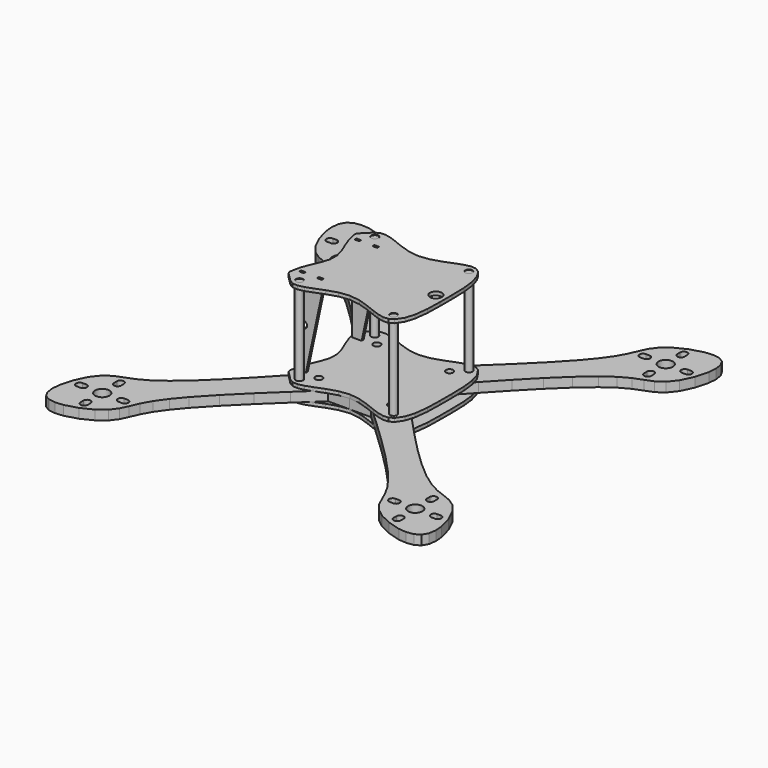
from build123d import *

# Parameters (mm, degrees)
F0_R      = 1.5
F0_R_2    = 3
F1_DEPTH  = 4
F3_DEPTH  = 4
F9_R      = 1.5
F10_DEPTH = 1.5
F12_R     = 1.5
F12_W     = 2
F12_H     = 1
F13_DEPTH = 1.5
F15_R     = 1.5
F15_W     = 2
F15_H     = 1
F15_R_2   = 2.5
F16_DEPTH = 1.5
F18_R     = 1.5
F19_DEPTH = 1
F21_DEPTH = 1
F23_R     = 1.5106239122
F24_DEPTH = 41.8
F23_R_2   = 1.5194161775
F23_R_3   = 1.519414421
F23_R_4   = 1.4934796866


# Not quite as in the source:
# - ends of sketch curves that miss each other by under 0.0002 mm in the source are joined


with BuildPart() as f1:
    # F0 (on Top) → F1 (new body)
    with BuildSketch(Plane.XY):
        Polygon((14.588631, -22.89682), (22.280861, -31.264773), (22.280861, -40.264773), (40.280861, -40.264773), (40.280861, -22.264773), (31.280861, -22.264773), (22.197863, -13.784713), (13.473396, -5.476525), (5.46599, 2.48792), (-1.465825, 9.93675), (-5.626846, 14.932085), (-8.891406, 19.497675), (-11.146676, 23.572215), (-12.706403, 27.176122), (-14.241022, 30.398156), (-16.431942, 33.329176), (-19.919393, 36.045885), (-24.80687, 38.450624), (-30.130665, 39.971349), (-33.488305, 40.264773), (-36.388928, 39.821389), (-38.572162, 38.503632), (-39.84702, 36.246807), (-40.280861, 33.257523), (-40.001152, 29.805519), (-38.522527, 24.349964), (-36.155436, 19.370567), (-33.323541, 15.755781), (-30.226835, 13.645808), (-26.791513, 12.264865), (-22.927057, 10.781282), (-18.549265, 8.401879), (-13.663209, 4.878131), (-7.22952, -0.641392), (-0.292414, -7.300286), (7.022254, -14.81371), align=None)
        with Locations((25.030861, -25.014773)):
            Circle(F0_R, mode=Mode.SUBTRACT)
        with Locations((20.513094, -20.497006)):
            Circle(F0_R, mode=Mode.SUBTRACT)
        with BuildLine():
            ThreePointArc((-26.922394, 17.438495), (-25.422394, 18.938495), (-23.922394, 17.438495))
            Line((-23.922394, 17.438495), (-23.922394, 15.938495))
            ThreePointArc((-23.922394, 15.938495), (-25.422394, 14.438495), (-26.922394, 15.938495))
            Line((-26.922394, 15.938495), (-26.922394, 17.438495))
        make_face(mode=Mode.SUBTRACT)
        with BuildLine():
            ThreePointArc((-34.922394, 23.938495), (-36.422394, 25.438495), (-34.922394, 26.938495))
            Line((-34.922394, 26.938495), (-33.422394, 26.938495))
            ThreePointArc((-33.422394, 26.938495), (-31.922394, 25.438495), (-33.422394, 23.938495))
            Line((-33.422394, 23.938495), (-34.922394, 23.938495))
        make_face(mode=Mode.SUBTRACT)
        with Locations((-25.427944, 25.444032)):
            Circle(F0_R_2, mode=Mode.SUBTRACT)
        with BuildLine():
            ThreePointArc((-23.922394, 33.438495), (-25.422394, 31.938495), (-26.922394, 33.438495))
            Line((-26.922394, 33.438495), (-26.922394, 34.938495))
            ThreePointArc((-26.922394, 34.938495), (-25.422394, 36.438495), (-23.922394, 34.938495))
            Line((-23.922394, 34.938495), (-23.922394, 33.438495))
        make_face(mode=Mode.SUBTRACT)
        with BuildLine():
            ThreePointArc((-15.922394, 26.938495), (-14.422394, 25.438495), (-15.922394, 23.938495))
            Line((-15.922394, 23.938495), (-17.422394, 23.938495))
            ThreePointArc((-17.422394, 23.938495), (-18.922394, 25.438495), (-17.422394, 26.938495))
            Line((-17.422394, 26.938495), (-15.922394, 26.938495))
        make_face(mode=Mode.SUBTRACT)
    extrude(amount=F1_DEPTH)


with BuildPart() as f1_1:
    # F2: moved
    add(f1.part.moved(Location((-40.3, 40.3, 0))))


with BuildPart() as f3:
    # F0 (on Top) → F3 (new body)
    with BuildSketch(Plane.XY):
        Polygon((14.588631, -22.89682), (22.280861, -31.264773), (22.280861, -40.264773), (40.280861, -40.264773), (40.280861, -22.264773), (31.280861, -22.264773), (22.197863, -13.784713), (13.473396, -5.476525), (5.46599, 2.48792), (-1.465825, 9.93675), (-5.626846, 14.932085), (-8.891406, 19.497675), (-11.146676, 23.572215), (-12.706403, 27.176122), (-14.241022, 30.398156), (-16.431942, 33.329176), (-19.919393, 36.045885), (-24.80687, 38.450624), (-30.130665, 39.971349), (-33.488305, 40.264773), (-36.388928, 39.821389), (-38.572162, 38.503632), (-39.84702, 36.246807), (-40.280861, 33.257523), (-40.001152, 29.805519), (-38.522527, 24.349964), (-36.155436, 19.370567), (-33.323541, 15.755781), (-30.226835, 13.645808), (-26.791513, 12.264865), (-22.927057, 10.781282), (-18.549265, 8.401879), (-13.663209, 4.878131), (-7.22952, -0.641392), (-0.292414, -7.300286), (7.022254, -14.81371), align=None)
        with Locations((25.030861, -25.014773)):
            Circle(F0_R, mode=Mode.SUBTRACT)
        with Locations((20.513094, -20.497006)):
            Circle(F0_R, mode=Mode.SUBTRACT)
        with BuildLine():
            ThreePointArc((-26.922394, 17.438495), (-25.422394, 18.938495), (-23.922394, 17.438495))
            Line((-23.922394, 17.438495), (-23.922394, 15.938495))
            ThreePointArc((-23.922394, 15.938495), (-25.422394, 14.438495), (-26.922394, 15.938495))
            Line((-26.922394, 15.938495), (-26.922394, 17.438495))
        make_face(mode=Mode.SUBTRACT)
        with BuildLine():
            ThreePointArc((-34.922394, 23.938495), (-36.422394, 25.438495), (-34.922394, 26.938495))
            Line((-34.922394, 26.938495), (-33.422394, 26.938495))
            ThreePointArc((-33.422394, 26.938495), (-31.922394, 25.438495), (-33.422394, 23.938495))
            Line((-33.422394, 23.938495), (-34.922394, 23.938495))
        make_face(mode=Mode.SUBTRACT)
        with Locations((-25.427944, 25.444032)):
            Circle(F0_R_2, mode=Mode.SUBTRACT)
        with BuildLine():
            ThreePointArc((-23.922394, 33.438495), (-25.422394, 31.938495), (-26.922394, 33.438495))
            Line((-26.922394, 33.438495), (-26.922394, 34.938495))
            ThreePointArc((-26.922394, 34.938495), (-25.422394, 36.438495), (-23.922394, 34.938495))
            Line((-23.922394, 34.938495), (-23.922394, 33.438495))
        make_face(mode=Mode.SUBTRACT)
        with BuildLine():
            ThreePointArc((-15.922394, 26.938495), (-14.422394, 25.438495), (-15.922394, 23.938495))
            Line((-15.922394, 23.938495), (-17.422394, 23.938495))
            ThreePointArc((-17.422394, 23.938495), (-18.922394, 25.438495), (-17.422394, 26.938495))
            Line((-17.422394, 26.938495), (-15.922394, 26.938495))
        make_face(mode=Mode.SUBTRACT)
    extrude(amount=F3_DEPTH)


with BuildPart() as f4_1:
    # F4: instance of F3
    add(f3.part.mirror(Plane.XZ))


with BuildPart() as f4_1_1:
    # F5: moved
    add(f4_1.part.moved(Location((-40.3, -40.3, 0))))


with BuildPart() as f7_1:
    # F7: instance of F1
    add(f1_1.part.mirror(Plane.YZ))


with BuildPart() as f8_1:
    # F8: instance of F7_1
    add(f7_1.part.mirror(Plane.XZ))


with BuildPart() as f10:
    # F9 (on Top) → F10 (new body)
    with BuildSketch(Plane.XY):
        with BuildLine():
            Line((-25.3842725429, -18.2968425442), (-21.776806, -21.90469))
            ThreePointArc((-21.776806, -21.90469), (-21.7695847524, -21.9118754367), (-21.7623269391, -21.9190239378))
            Line((-21.7623269391, -21.9190239378), (-20.001088, -22.921175))
            Line((-20.001088, -22.921175), (-17.861866, -23.035324))
            Line((-17.861866, -23.035324), (-15.372177, -22.484303))
            Line((-15.372177, -22.484303), (-12.607263, -21.500754))
            Line((-12.607263, -21.500754), (-8.588488, -19.927774))
            Line((-8.588488, -19.927774), (-4.3106, -18.572828))
            Line((-4.3106, -18.572828), (0.094871, -17.999903))
            Line((0.094871, -17.999903), (4.497054, -18.584621))
            Line((4.497054, -18.584621), (8.767715, -19.949316))
            Line((8.767715, -19.949316), (12.779279, -21.528046))
            Line((12.779279, -21.528046), (15.541174, -22.512101))
            Line((15.541174, -22.512101), (18.031746, -23.059449))
            Line((18.031746, -23.059449), (20.197174, -22.931331))
            Line((20.197174, -22.931331), (21.983635, -21.88899))
            Line((21.983635, -21.88899), (23.940328, -18.98249))
            Line((23.940328, -18.98249), (25.122837, -15.218566))
            Line((25.122837, -15.218566), (25.815172, -9.515305))
            Line((25.815172, -9.515305), (25.969817, -3.186776))
            Line((25.969817, -3.186776), (25.969969, 3.339753))
            Line((25.969969, 3.339753), (25.807978, 9.644786))
            Line((25.807978, 9.644786), (25.256208, 14.514056))
            Line((25.256208, 14.514056), (24.06386, 18.675831))
            Line((24.06386, 18.675831), (21.985337, 21.878655))
            ThreePointArc((21.985337, 21.878655), (21.9798580505, 21.8841874891), (21.9743579768, 21.8896989767))
            Line((21.9743579768, 21.8896989767), (20.209215, 22.909511))
            Line((20.209215, 22.909511), (18.056913, 23.026143))
            Line((18.056913, 23.026143), (15.568049, 22.474392))
            Line((15.568049, 22.474392), (12.802409, 21.490951))
            Line((12.802409, 21.490951), (8.781129, 19.919049))
            Line((8.781129, 19.919049), (4.50007, 18.565781))
            Line((4.50007, 18.565781), (0.091958, 17.994625))
            Line((0.091958, 17.994625), (-4.31142, 18.580902))
            Line((-4.31142, 18.580902), (-8.582017, 19.946966))
            Line((-8.582017, 19.946966), (-12.592724, 21.526836))
            Line((-12.592724, 21.526836), (-15.353738, 22.511578))
            Line((-15.353738, 22.511578), (-17.843441, 23.059449))
            Line((-17.843441, 23.059449), (-19.987611, 22.937283))
            Line((-19.987611, 22.937283), (-21.761576, 21.921992))
            ThreePointArc((-21.761576, 21.921992), (-21.7690321095, 21.9146523137), (-21.7764495624, 21.9072735624))
            Line((-21.7764495624, 21.9072735624), (-25.300048, 18.383676))
            ThreePointArc((-25.300048, 18.383676), (-25.7704478547, 17.6389622754), (-25.8752922762, 16.7643869715))
            Line((-25.8752922762, 16.7643869715), (-24.974945, 12.734506))
            Line((-24.974945, 12.734506), (-23.49499, 8.878377))
            Line((-23.49499, 8.878377), (-21.991471, 5.171737))
            Line((-21.991471, 5.171737), (-21.020436, 1.590323))
            Line((-21.020436, 1.590323), (-21.107345, -1.893192))
            Line((-21.107345, -1.893192), (-22.181047, -5.300749))
            Line((-22.181047, -5.300749), (-23.708361, -8.823601))
            Line((-23.708361, -8.823601), (-25.149676, -12.591593))
            Line((-25.149676, -12.591593), (-25.965377, -16.734569))
            Line((-25.965377, -16.734569), (-25.968026, -16.794603))
            ThreePointArc((-25.968026, -16.794603), (-25.8343859413, -17.606587539), (-25.3851102659, -18.2960292498))
            Line((-25.3851102659, -18.2960292498), (-25.3842725429, -18.2968425442))
        make_face()
        with Locations((-19.630301, -19.80957)):
            Circle(F9_R, mode=Mode.SUBTRACT)
        with Locations((-15.155452, -15.249903)):
            Circle(F9_R, mode=Mode.SUBTRACT)
        with Locations((19.862315, -19.76767)):
            Circle(F9_R, mode=Mode.SUBTRACT)
        with Locations((15.344548, -15.249903)):
            Circle(F9_R, mode=Mode.SUBTRACT)
        with Locations((-15.155452, 15.250097)):
            Circle(F9_R, mode=Mode.SUBTRACT)
        with Locations((-19.673219, 19.767864)):
            Circle(F9_R, mode=Mode.SUBTRACT)
        with Locations((15.344548, 15.250097)):
            Circle(F9_R, mode=Mode.SUBTRACT)
        with Locations((19.862315, 19.767864)):
            Circle(F9_R, mode=Mode.SUBTRACT)
    extrude(amount=F10_DEPTH)


with BuildPart() as f10_1:
    # F11: moved
    add(f10.part.moved(Location((0, 0, -1.5))))


with BuildPart() as f13:
    # F12 (on Top) → F13 (new body)
    with BuildSketch(Plane.XY):
        with BuildLine():
            Line((-25.3842725429, -18.2968425442), (-21.776806, -21.90469))
            ThreePointArc((-21.776806, -21.90469), (-21.7695847524, -21.9118754367), (-21.7623269391, -21.9190239378))
            Line((-21.7623269391, -21.9190239378), (-20.001088, -22.921175))
            Line((-20.001088, -22.921175), (-17.861866, -23.035324))
            Line((-17.861866, -23.035324), (-15.372177, -22.484303))
            Line((-15.372177, -22.484303), (-12.607263, -21.500754))
            Line((-12.607263, -21.500754), (-8.588488, -19.927774))
            Line((-8.588488, -19.927774), (-4.3106, -18.572828))
            Line((-4.3106, -18.572828), (0.094871, -17.999903))
            Line((0.094871, -17.999903), (4.497054, -18.584621))
            Line((4.497054, -18.584621), (8.767715, -19.949316))
            Line((8.767715, -19.949316), (12.779279, -21.528046))
            Line((12.779279, -21.528046), (15.541174, -22.512101))
            Line((15.541174, -22.512101), (18.031746, -23.059449))
            Line((18.031746, -23.059449), (20.197174, -22.931331))
            Line((20.197174, -22.931331), (21.983635, -21.88899))
            Line((21.983635, -21.88899), (23.940328, -18.98249))
            Line((23.940328, -18.98249), (25.122837, -15.218566))
            Line((25.122837, -15.218566), (25.815172, -9.515305))
            Line((25.815172, -9.515305), (25.969817, -3.186776))
            Line((25.969817, -3.186776), (25.969969, 3.339753))
            Line((25.969969, 3.339753), (25.807978, 9.644786))
            Line((25.807978, 9.644786), (25.256208, 14.514056))
            Line((25.256208, 14.514056), (24.06386, 18.675831))
            Line((24.06386, 18.675831), (21.985337, 21.878655))
            ThreePointArc((21.985337, 21.878655), (21.9798580505, 21.8841874891), (21.9743579768, 21.8896989767))
            Line((21.9743579768, 21.8896989767), (20.209215, 22.909511))
            Line((20.209215, 22.909511), (18.056913, 23.026143))
            Line((18.056913, 23.026143), (15.568049, 22.474392))
            Line((15.568049, 22.474392), (12.802409, 21.490951))
            Line((12.802409, 21.490951), (8.781129, 19.919049))
            Line((8.781129, 19.919049), (4.50007, 18.565781))
            Line((4.50007, 18.565781), (0.091958, 17.994625))
            Line((0.091958, 17.994625), (-4.31142, 18.580902))
            Line((-4.31142, 18.580902), (-8.582017, 19.946966))
            Line((-8.582017, 19.946966), (-12.592724, 21.526836))
            Line((-12.592724, 21.526836), (-15.353738, 22.511578))
            Line((-15.353738, 22.511578), (-17.843441, 23.059449))
            Line((-17.843441, 23.059449), (-19.987611, 22.937283))
            Line((-19.987611, 22.937283), (-21.761576, 21.921992))
            ThreePointArc((-21.761576, 21.921992), (-21.7690321095, 21.9146523137), (-21.7764495624, 21.9072735624))
            Line((-21.7764495624, 21.9072735624), (-25.300048, 18.383676))
            ThreePointArc((-25.300048, 18.383676), (-25.7704478547, 17.6389622754), (-25.8752922762, 16.7643869715))
            Line((-25.8752922762, 16.7643869715), (-24.974945, 12.734506))
            Line((-24.974945, 12.734506), (-23.49499, 8.878377))
            Line((-23.49499, 8.878377), (-21.991471, 5.171737))
            Line((-21.991471, 5.171737), (-21.020436, 1.590323))
            Line((-21.020436, 1.590323), (-21.107345, -1.893192))
            Line((-21.107345, -1.893192), (-22.181047, -5.300749))
            Line((-22.181047, -5.300749), (-23.708361, -8.823601))
            Line((-23.708361, -8.823601), (-25.149676, -12.591593))
            Line((-25.149676, -12.591593), (-25.965377, -16.734569))
            Line((-25.965377, -16.734569), (-25.968026, -16.794603))
            ThreePointArc((-25.968026, -16.794603), (-25.8343859413, -17.606587539), (-25.3851102659, -18.2960292498))
            Line((-25.3851102659, -18.2960292498), (-25.3842725429, -18.2968425442))
        make_face()
        with Locations((-19.630301, -19.80957)):
            Circle(F12_R, mode=Mode.SUBTRACT)
        with Locations((-22.655452, -14.499902)):
            Rectangle(F12_W, F12_H, mode=Mode.SUBTRACT)
        with Locations((-15.155452, -15.249903)):
            Circle(F12_R, mode=Mode.SUBTRACT)
        with Locations((19.862315, -19.76767)):
            Circle(F12_R, mode=Mode.SUBTRACT)
        with Locations((15.344548, -15.249903)):
            Circle(F12_R, mode=Mode.SUBTRACT)
        with Locations((-22.655452, 14.600097)):
            Rectangle(F12_W, F12_H, mode=Mode.SUBTRACT)
        with Locations((-15.155452, 15.250097)):
            Circle(F12_R, mode=Mode.SUBTRACT)
        with Locations((-19.673219, 19.767864)):
            Circle(F12_R, mode=Mode.SUBTRACT)
        with Locations((15.344548, 15.250097)):
            Circle(F12_R, mode=Mode.SUBTRACT)
        with Locations((19.862315, 19.767864)):
            Circle(F12_R, mode=Mode.SUBTRACT)
    extrude(amount=F13_DEPTH)


with BuildPart() as f13_1:
    # F14: moved
    add(f13.part.moved(Location((0, 0, 4))))


with BuildPart() as f16:
    # F15 (on Top) → F16 (new body)
    with BuildSketch(Plane.XY):
        with BuildLine():
            Line((-25.3842725429, -18.2968425442), (-21.776806, -21.90469))
            ThreePointArc((-21.776806, -21.90469), (-21.7695847524, -21.9118754367), (-21.7623269391, -21.9190239378))
            Line((-21.7623269391, -21.9190239378), (-20.001088, -22.921175))
            Line((-20.001088, -22.921175), (-17.861866, -23.035324))
            Line((-17.861866, -23.035324), (-15.372177, -22.484303))
            Line((-15.372177, -22.484303), (-12.607263, -21.500754))
            Line((-12.607263, -21.500754), (-8.588488, -19.927774))
            Line((-8.588488, -19.927774), (-4.3106, -18.572828))
            Line((-4.3106, -18.572828), (0.094871, -17.999903))
            Line((0.094871, -17.999903), (4.497054, -18.584621))
            Line((4.497054, -18.584621), (8.767715, -19.949316))
            Line((8.767715, -19.949316), (12.779279, -21.528046))
            Line((12.779279, -21.528046), (15.541174, -22.512101))
            Line((15.541174, -22.512101), (18.031746, -23.059449))
            Line((18.031746, -23.059449), (20.197174, -22.931331))
            Line((20.197174, -22.931331), (21.983635, -21.88899))
            Line((21.983635, -21.88899), (23.940328, -18.98249))
            Line((23.940328, -18.98249), (25.122837, -15.218566))
            Line((25.122837, -15.218566), (25.815172, -9.515305))
            Line((25.815172, -9.515305), (25.969817, -3.186776))
            Line((25.969817, -3.186776), (25.969969, 3.339753))
            Line((25.969969, 3.339753), (25.807978, 9.644786))
            Line((25.807978, 9.644786), (25.256208, 14.514056))
            Line((25.256208, 14.514056), (24.06386, 18.675831))
            Line((24.06386, 18.675831), (22.2375132143, 21.6685608029))
            Line((22.2375132143, 21.6685608029), (20.209215, 22.909511))
            Line((20.209215, 22.909511), (18.056913, 23.026143))
            Line((18.056913, 23.026143), (15.568049, 22.474392))
            Line((15.568049, 22.474392), (12.802409, 21.490951))
            Line((12.802409, 21.490951), (8.781129, 19.919049))
            Line((8.781129, 19.919049), (4.50007, 18.565781))
            Line((4.50007, 18.565781), (0.091958, 17.994625))
            Line((0.091958, 17.994625), (-4.31142, 18.580902))
            Line((-4.31142, 18.580902), (-8.582017, 19.946966))
            Line((-8.582017, 19.946966), (-12.592724, 21.526836))
            Line((-12.592724, 21.526836), (-15.353738, 22.511578))
            Line((-15.353738, 22.511578), (-17.843441, 23.059449))
            Line((-17.843441, 23.059449), (-19.987611, 22.937283))
            Line((-19.987611, 22.937283), (-21.761576, 21.921992))
            ThreePointArc((-21.761576, 21.921992), (-21.7690321095, 21.9146523137), (-21.7764495624, 21.9072735624))
            Line((-21.7764495624, 21.9072735624), (-25.300048, 18.383676))
            ThreePointArc((-25.300048, 18.383676), (-25.7704478547, 17.6389622754), (-25.8752922762, 16.7643869715))
            Line((-25.8752922762, 16.7643869715), (-24.974945, 12.734506))
            Line((-24.974945, 12.734506), (-23.49499, 8.878377))
            Line((-23.49499, 8.878377), (-21.991471, 5.171737))
            Line((-21.991471, 5.171737), (-21.020436, 1.590323))
            Line((-21.020436, 1.590323), (-21.107345, -1.893192))
            Line((-21.107345, -1.893192), (-22.181047, -5.300749))
            Line((-22.181047, -5.300749), (-23.708361, -8.823601))
            Line((-23.708361, -8.823601), (-25.149676, -12.591593))
            Line((-25.149676, -12.591593), (-25.965377, -16.734569))
            Line((-25.965377, -16.734569), (-25.968026, -16.794603))
            ThreePointArc((-25.968026, -16.794603), (-25.8343859413, -17.606587539), (-25.3851102659, -18.2960292498))
            Line((-25.3851102659, -18.2960292498), (-25.3842725429, -18.2968425442))
        make_face()
        with Locations((-19.630301, -19.80957)):
            Circle(F15_R, mode=Mode.SUBTRACT)
        with Locations((-22.655452, -14.499902)):
            Rectangle(F15_W, F15_H, mode=Mode.SUBTRACT)
        with Locations((-15.155479, -14.499902)):
            Rectangle(F15_W, F15_H, mode=Mode.SUBTRACT)
        with Locations((19.862315, -19.76767)):
            Circle(F15_R, mode=Mode.SUBTRACT)
        with Locations((-22.655452, 14.600097)):
            Rectangle(F15_W, F15_H, mode=Mode.SUBTRACT)
        with Locations((-15.155479, 14.600097)):
            Rectangle(F15_W, F15_H, mode=Mode.SUBTRACT)
        with Locations((-19.673219, 19.767864)):
            Circle(F15_R, mode=Mode.SUBTRACT)
        with Locations((21.776255, 9.7e-05)):
            Circle(F15_R_2, mode=Mode.SUBTRACT)
        with Locations((19.862315, 19.767864)):
            Circle(F15_R, mode=Mode.SUBTRACT)
    extrude(amount=F16_DEPTH)


with BuildPart() as f16_1:
    # F17: moved
    add(f16.part.moved(Location((0, 0, 40.5))))


with BuildPart() as f19:
    # F18 (on Front) → F19 (new body)
    with BuildSketch(Plane.XZ):
        Polygon((-4.75, 17.5), (-5.75, 17.5), (-5.75, -17.5), (-4.75, -17.5), (-4.75, -18.5), (-2.75, -18.5), (-2.75, -17.5), (-1.75, -17.5), (5.75, 17.5), (4.75, 17.5), (4.75, 18.5), (2.75, 18.5), (2.75, 17.5), (-2.75, 17.5), (-2.75, 18.5), (-4.75, 18.5), align=None)
        with Locations((-2.75, 0)):
            Circle(F18_R, mode=Mode.SUBTRACT)
    extrude(amount=F19_DEPTH)


with BuildPart() as f19_1:
    # F20: moved
    add(f19.part.moved(Location((-19.03, -14.04, 23.01))))


with BuildPart() as f21:
    # F18 (on Front) → F21 (new body)
    with BuildSketch(Plane.XZ):
        Polygon((-4.75, 17.5), (-5.75, 17.5), (-5.75, -17.5), (-4.75, -17.5), (-4.75, -18.5), (-2.75, -18.5), (-2.75, -17.5), (-1.75, -17.5), (5.75, 17.5), (4.75, 17.5), (4.75, 18.5), (2.75, 18.5), (2.75, 17.5), (-2.75, 17.5), (-2.75, 18.5), (-4.75, 18.5), align=None)
        with Locations((-2.75, 0)):
            Circle(F18_R, mode=Mode.SUBTRACT)
    extrude(amount=F21_DEPTH)


with BuildPart() as f21_1:
    # F22: moved
    add(f21.part.moved(Location((-18.9, 15.1, 23.03))))


with BuildPart() as f24:
    # F23 (on Top) → F24 (new body)
    with BuildSketch(Plane.XY):
        with Locations((-19.7049248964, -19.8188405484)):
            Circle(F23_R)
    extrude(amount=F24_DEPTH)


with BuildPart() as f24b:
    # F23 (on Top) → F24, piece 2 (new body)
    with BuildSketch(Plane.XY):
        with Locations((19.7811666876, -19.7767019272)):
            Circle(F23_R_2)
    extrude(amount=F24_DEPTH)


with BuildPart() as f24c:
    # F23 (on Top) → F24, piece 3 (new body)
    with BuildSketch(Plane.XY):
        with Locations((19.8654476553, 19.7515301406)):
            Circle(F23_R_3)
    extrude(amount=F24_DEPTH)


with BuildPart() as f24d:
    # F23 (on Top) → F24, piece 4 (new body)
    with BuildSketch(Plane.XY):
        with Locations((-19.7470672429, 19.7515301406)):
            Circle(F23_R_4)
    extrude(amount=F24_DEPTH)


solid = Compound([f1_1.part, f4_1_1.part, f7_1.part, f8_1.part, f10_1.part, f13_1.part, f16_1.part, f19_1.part, f21_1.part, f24.part, f24b.part, f24c.part, f24d.part])
